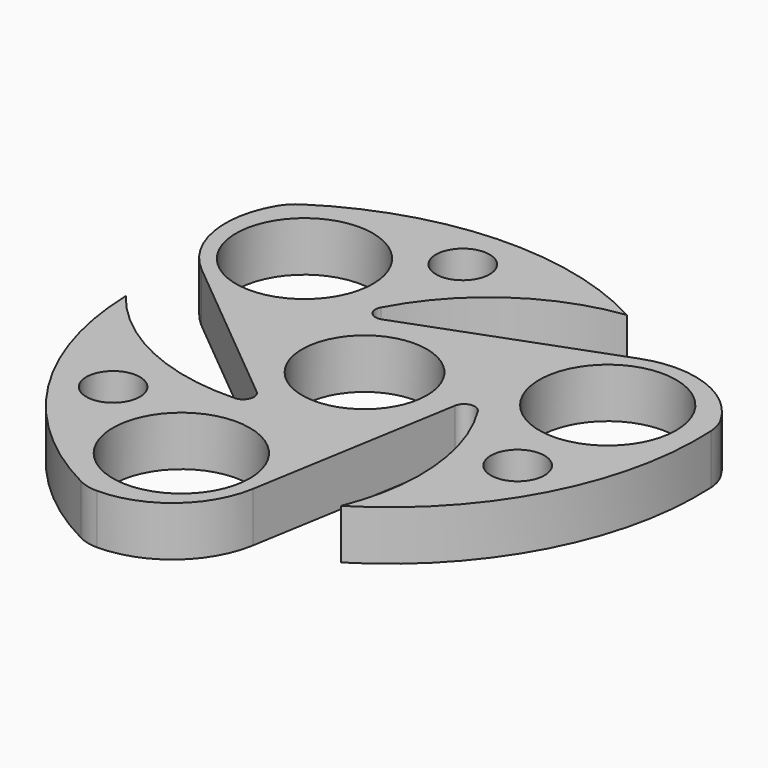
from build123d import *

# Parameters (mm, degrees)
F0_R     = 12.1158
F0_R_2   = 4.7498
F0_R_3   = 11.049
F1_DEPTH = 8.8138
F2_R     = 7.62


# Not quite as in the source:
# - ends of sketch curves that miss each other by under 0.0002 mm in the source are joined


with BuildPart() as f1:
    # F0 (on Top) → F1 (new body)
    with BuildSketch(Plane.XY):
        with BuildLine():
            ThreePointArc((22.4249021167, -33.2598383611), (42.5511926564, -11.3994547245), (48.2521252698, 17.762906479))
            ThreePointArc((48.2521252698, 17.762906479), (39.4932996014, 26.5789641765), (27.0699823404, 26.8969085886))
            Line((27.0699823404, 26.8969085886), (-8.0010006819, 13.8581388051))
            ThreePointArc((-8.0010006819, 13.8581388051), (-10.1044657967, 14.3898463988), (-10.3558611613, 16.5448588871))
            ThreePointArc((-10.3558611613, 16.5448588871), (1.2618519363, 29.6731834096), (17.5914130917, 36.0504551503))
            ThreePointArc((17.5914130917, 36.0504551503), (-11.4033797439, 42.5501422233), (-39.5091916872, 32.90611409))
            ThreePointArc((-39.5091916872, 32.90611409), (-42.7647087802, 20.9127197051), (-36.8283980876, 9.9948391518))
            Line((-36.8283980876, 9.9948391518), (-8.0010006819, -13.8581382646))
            ThreePointArc((-8.0010006819, -13.8581382646), (-7.409740408, -15.9456462868), (-9.1503382861, -17.2408673032))
            ThreePointArc((-9.1503382861, -17.2408673032), (-26.3286573805, -13.743794888), (-40.0163172925, -2.7906159651))
            ThreePointArc((-40.0163172925, -2.7906159651), (-31.1478149966, -31.1506866748), (-8.7429356667, -50.669019745))
            ThreePointArc((-8.7429356667, -50.669019745), (3.2714070948, -47.4916830576), (9.7584136631, -36.8917469163))
            Line((9.7584136631, -36.8917469163), (16.0019992774, 2.702e-07))
            ThreePointArc((16.0019992774, 2.702e-07), (17.514204114, 1.5558007108), (19.5061973633, 0.6960092401))
            ThreePointArc((19.5061973633, 0.6960092401), (25.0668033601, -15.9293876975), (22.4249021167, -33.2598383611))
        make_face()
        with Locations((-4.651045185, -34.7045873419)):
            Circle(F0_R, mode=Mode.SUBTRACT)
        with Locations((-24.3930550349, -25.1201008156)):
            Circle(F0_R_2, mode=Mode.SUBTRACT)
        with Locations((33.9511726837, -8.5649542264)):
            Circle(F0_R_2, mode=Mode.SUBTRACT)
        Circle(F0_R_3, mode=Mode.SUBTRACT)
        with Locations((-27.7295329099, 21.3802167818)):
            Circle(F0_R, mode=Mode.SUBTRACT)
        with Locations((-9.5581186852, 33.6850558475)):
            Circle(F0_R_2, mode=Mode.SUBTRACT)
        with Locations((32.3805760108, 13.3243713841)):
            Circle(F0_R, mode=Mode.SUBTRACT)
    extrude(amount=F1_DEPTH)

    # F2
    f2_edges = [f1.edges().sort_by_distance(p)[0] for p in [
        (-39.509192, 32.906114, 4.4069),
        (48.252125, 17.762906, 4.4069),
        (-8.742936, -50.66902, 4.4069),
    ]]
    fillet(f2_edges, radius=F2_R)


solid = f1.part
